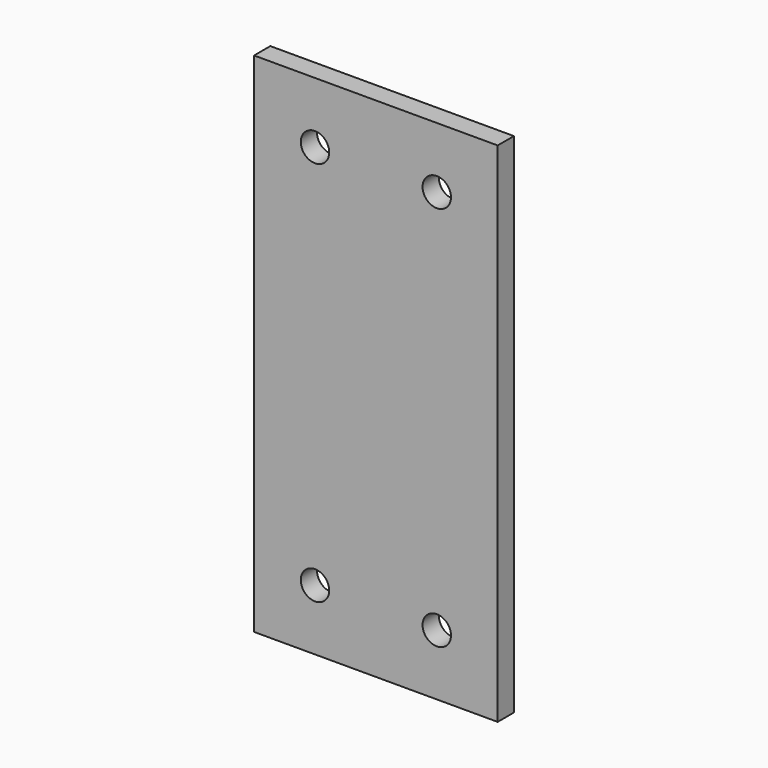
from build123d import *

# Parameters (mm, degrees)
F0_W     = 120
F0_H     = 250
F0_R     = 7
F1_DEPTH = 10


# Not quite as in the source:
# - a feature names something its author has since deleted; it is built from what else it names


with BuildPart() as f1:
    # F0 (on Front) → F1 (new body)
    with BuildSketch(Plane.XZ):
        Rectangle(F0_W, F0_H)
        with Locations((-30, -95)):
            Circle(F0_R, mode=Mode.SUBTRACT)
        with Locations((30, -95)):
            Circle(F0_R, mode=Mode.SUBTRACT)
        with Locations((-30, 95)):
            Circle(F0_R, mode=Mode.SUBTRACT)
        with Locations((30, 95)):
            Circle(F0_R, mode=Mode.SUBTRACT)
    extrude(amount=F1_DEPTH)


solid = f1.part
